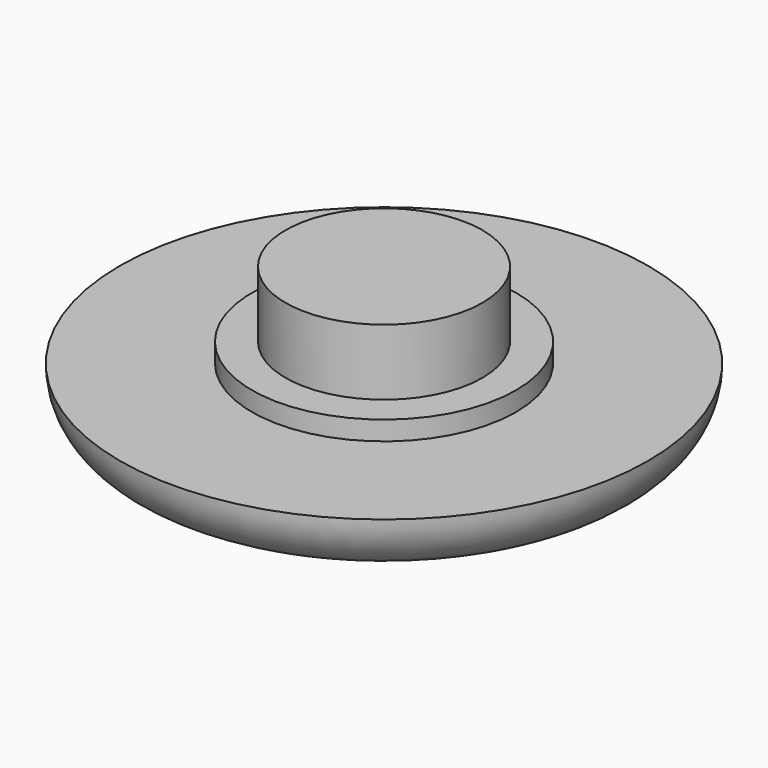
from build123d import *

# Parameters (mm, degrees)
F0_R      = 11
F0_R_2    = 5.5
F1_DEPTH  = 2.5
F0_R_3    = 4.1
F2_DEPTH  = 3.3
F3_DEPTH  = 6.05
F4_R      = 2.49999
F7_W      = 0.7752131331
F7_H      = 1.8432312268
F7_H_2    = 1.8120306982
F8_DEPTH  = 1
F9_W      = 0.005
F9_H      = 0.6400108426
F10_DEPTH = 0.1


# Not quite as in the source:
# - a fillet or chamfer is up to 0.001 mm smaller than in the source, because OpenCascade refuses the exact size


with BuildPart() as f1:
    # F0 (on Top) → F1 (new body)
    with BuildSketch(Plane.XY):
        Circle(F0_R)
        Circle(F0_R_2, mode=Mode.SUBTRACT)
    extrude(amount=F1_DEPTH)

    # F0 (on Top) → F2 (join, through all)
    with BuildSketch(Plane.XY):
        Circle(F0_R_2)
        Circle(F0_R_3, mode=Mode.SUBTRACT)
    extrude(amount=F2_DEPTH)

    # F0 (on Top) → F3 (join, through all)
    with BuildSketch(Plane.XY):
        Circle(F0_R_3)
    extrude(amount=F3_DEPTH)

    # F4 (radius 2.5 in the source; OpenCascade refuses exactly that, so slightly less here)
    f4_edges = [f1.edges().sort_by_distance(p)[0] for p in [
        (-11, 0, 0),
    ]]
    fillet(f4_edges, radius=F4_R)

    # F7 (on face) → F8 (cut)
    with BuildSketch(Plane(origin=(0, 0, 0), x_dir=(1, 0, 0), z_dir=(0, 0, -1))):
        with BuildLine():
            Line((-7.8377327815, 1.8120306982), (-7.8377327815, 0))
            Line((-7.8377327815, 0), (-7.0625196484, 0))
            Line((-7.0625196484, 0), (-7.0625196484, 1.1768199369))
            Line((-7.0625196484, 1.1768199369), (-6.6505126685, 1.1768199369))
            add(Edge.make_bspline(
                [(-5.6104951692, 0), (-5.6108483761, 1.1768199369), (-6.6505126685, 1.1768199369)],
                knots=[0.0003397316, 0.0003397316, 0.0003397316, 1, 1, 1], degree=2))
            Line((-5.6104951692, 0), (-4.8049398646, 0))
            add(Edge.make_bspline(
                [(-4.804881401, 0.0192003253), (-4.804881401, 0.0095761402), (-4.8049398646, 0)],
                knots=[0, 0, 0, 0.010664918, 0.010664918, 0.010664918], degree=2))
            add(Edge.make_bspline(
                [(-5.3000897905, 1.339622695), (-4.804881401, 0.8672146918), (-4.804881401, 0.0192003253)],
                knots=[0, 0, 0, 1, 1, 1], degree=2))
            add(Edge.make_bspline(
                [(-6.6905133461, 1.8120306982), (-5.79529818, 1.8120306982), (-5.3000897905, 1.339622695)],
                knots=[0, 0, 0, 1, 1, 1], degree=2))
            Line((-6.6905133461, 1.8120306982), (-7.8377327815, 1.8120306982))
        make_face()
        with BuildLine():
            Line((-7.0625196484, 0), (-7.8377327815, 0))
            Line((-7.8377327815, 0), (-7.8377327815, -1.8432312268))
            Line((-7.8377327815, -1.8432312268), (-6.8025152436, -1.8432312268))
            add(Edge.make_bspline(
                [(-5.318890109, -1.3632230948), (-5.832898817, -1.8432312268), (-6.8025152436, -1.8432312268)],
                knots=[0, 0, 0, 1, 1, 1], degree=2))
            add(Edge.make_bspline(
                [(-4.8049398646, 0), (-4.8103632617, -0.8883342102), (-5.318890109, -1.3632230948)],
                knots=[0.010664918, 0.010664918, 0.010664918, 1, 1, 1], degree=2))
            Line((-4.8049398646, 0), (-5.6104951692, 0))
            add(Edge.make_bspline(
                [(-5.6104950492, -0.0008000136), (-5.6104950492, -0.0003999388), (-5.6104951692, 0)],
                knots=[0, 0, 0, 0.0003397316, 0.0003397316, 0.0003397316], degree=2))
            add(Edge.make_bspline(
                [(-6.7305140238, -1.2032203841), (-5.6104950492, -1.2032203841), (-5.6104950492, -0.0008000136)],
                knots=[0, 0, 0, 1, 1, 1], degree=2))
            Line((-6.7305140238, -1.2032203841), (-7.0625196484, -1.2032203841))
            Line((-7.0625196484, -1.2032203841), (-7.0625196484, 0))
        make_face()
        Polygon((6.1985050109, 1.1672197742), (6.1985050109, 0), (6.973718144, 0), (6.973718144, 1.1672197742), (7.9657349501, 1.1672197742), (7.9657349501, 1.8120306982), (5.2056881912, 1.8120306982), (5.2056881912, 1.1672197742), align=None)
        with Locations((6.5861115774, -0.9216156134)):
            Rectangle(F7_W, F7_H)
        Polygon((3.2336547824, 1.1672197742), (3.2336547824, 0), (4.0088679155, 0), (4.0088679155, 1.1672197742), (5.0008847216, 1.1672197742), (5.0008847216, 1.8120306982), (2.2408379628, 1.8120306982), (2.2408379628, 1.1672197742), align=None)
        with Locations((3.6212613489, -0.9216156134)):
            Rectangle(F7_W, F7_H)
        with Locations((1.2908218682, 0.9060153491)):
            Rectangle(F7_W, F7_H_2)
        with Locations((1.2908218682, -0.9216156134)):
            Rectangle(F7_W, F7_H)
        Polygon((-4.5072763592, 1.8120306982), (-4.044849615, 0), (-3.3198281749, 0), (-3.7448634429, 1.8120306982), align=None)
        with BuildLine():
            Line((-3.3198281749, 0), (-4.044849615, 0))
            Line((-4.044849615, 0), (-3.5744605561, -1.8432312268))
            Line((-3.5744605561, -1.8432312268), (-2.6944456475, -1.8432312268))
            Line((-2.6944456475, -1.8432312268), (-2.2209338662, 0))
            Line((-2.2209338662, 0), (-2.868251717, 0))
            Line((-2.868251717, 0), (-2.9296496321, -0.2360039982))
            add(Edge.make_bspline(
                [(-3.0308513466, -0.6996118523), (-2.9768504318, -0.4008067902), (-2.9296496321, -0.2360039982)],
                knots=[0, 0, 0, 1, 1, 1], degree=2))
            add(Edge.make_bspline(
                [(-3.100052519, -1.140819327), (-3.0848522615, -0.9984169145), (-3.0308513466, -0.6996118523)],
                knots=[0, 0, 0, 1, 1, 1], degree=2))
            add(Edge.make_bspline(
                [(-3.2768555143, -0.1832031037), (-3.1544534406, -0.736012469), (-3.100052519, -1.140819327)],
                knots=[0, 0, 0, 1, 1, 1], degree=2))
            Line((-3.2768555143, -0.1832031037), (-3.3198281749, 0))
        make_face()
        with BuildLine():
            Line((-2.868251717, 0), (-3.3198281749, 0))
            Line((-3.3198281749, 0), (-3.2768555143, -0.1832031037))
            add(Edge.make_bspline(
                [(-3.2768555143, -0.1832031037), (-3.1544534406, -0.736012469), (-3.100052519, -1.140819327)],
                knots=[0, 0, 0, 1, 1, 1], degree=2))
            add(Edge.make_bspline(
                [(-3.100052519, -1.140819327), (-3.0848522615, -0.9984169145), (-3.0308513466, -0.6996118523)],
                knots=[0, 0, 0, 1, 1, 1], degree=2))
            add(Edge.make_bspline(
                [(-3.0308513466, -0.6996118523), (-2.9768504318, -0.4008067902), (-2.9296496321, -0.2360039982)],
                knots=[0, 0, 0, 1, 1, 1], degree=2))
            Line((-2.9296496321, -0.2360039982), (-2.868251717, 0))
        make_face()
        with BuildLine():
            Line((-2.3968406056, 1.8120306982), (-2.868251717, 0))
            Line((-2.868251717, 0), (-2.2209338662, 0))
            Line((-2.2209338662, 0), (-2.2024373122, 0.0720012198))
            add(Edge.make_bspline(
                [(-2.10963574, 0.4980084369), (-2.1696367565, 0.1992033748), (-2.2024373122, 0.0720012198)],
                knots=[0, 0, 0, 1, 1, 1], degree=2))
            add(Edge.make_bspline(
                [(-2.034434466, 0.9320157896), (-2.0496347235, 0.7968134991), (-2.10963574, 0.4980084369)],
                knots=[0, 0, 0, 1, 1, 1], degree=2))
            add(Edge.make_bspline(
                [(-1.9584331784, 0.5004084776), (-2.0248343034, 0.8216139192), (-2.034434466, 0.9320157896)],
                knots=[0, 0, 0, 1, 1, 1], degree=2))
            add(Edge.make_bspline(
                [(-1.8648315927, 0.0768013011), (-1.8920320535, 0.1792030359), (-1.9584331784, 0.5004084776)],
                knots=[0, 0, 0, 1, 1, 1], degree=2))
            Line((-1.8648315927, 0.0768013011), (-1.8450232571, 0))
            Line((-1.8450232571, 0), (-1.1934170931, 0))
            Line((-1.1934170931, 0), (-1.6648282044, 1.8120306982))
            Line((-1.6648282044, 1.8120306982), (-2.3968406056, 1.8120306982))
        make_face()
        with BuildLine():
            Line((-2.2024373122, 0.0720012198), (-2.2209338662, 0))
            Line((-2.2209338662, 0), (-1.8450232571, 0))
            Line((-1.8450232571, 0), (-1.8648315927, 0.0768013011))
            add(Edge.make_bspline(
                [(-1.8648315927, 0.0768013011), (-1.8920320535, 0.1792030359), (-1.9584331784, 0.5004084776)],
                knots=[0, 0, 0, 1, 1, 1], degree=2))
            add(Edge.make_bspline(
                [(-1.9584331784, 0.5004084776), (-2.0248343034, 0.8216139192), (-2.034434466, 0.9320157896)],
                knots=[0, 0, 0, 1, 1, 1], degree=2))
            add(Edge.make_bspline(
                [(-2.034434466, 0.9320157896), (-2.0496347235, 0.7968134991), (-2.10963574, 0.4980084369)],
                knots=[0, 0, 0, 1, 1, 1], degree=2))
            add(Edge.make_bspline(
                [(-2.10963574, 0.4980084369), (-2.1696367565, 0.1992033748), (-2.2024373122, 0.0720012198)],
                knots=[0, 0, 0, 1, 1, 1], degree=2))
        make_face()
        with BuildLine():
            Line((-1.1934170931, 0), (-1.8450232571, 0))
            Line((-1.8450232571, 0), (-1.3696232032, -1.8432312268))
            Line((-1.3696232032, -1.8432312268), (-0.487208254, -1.8432312268))
            Line((-0.487208254, -1.8432312268), (-0.0180294584, 0))
            Line((-0.0180294584, 0), (-0.7421344653, 0))
            Line((-0.7421344653, 0), (-0.7848132958, -0.1832031037))
            add(Edge.make_bspline(
                [(-0.8848149899, -0.6544110866), (-0.8296140548, -0.3632061532), (-0.7848132958, -0.1832031037)],
                knots=[0, 0, 0, 1, 1, 1], degree=2))
            add(Edge.make_bspline(
                [(-0.9648163453, -1.140819327), (-0.9400159251, -0.94561602), (-0.8848149899, -0.6544110866)],
                knots=[0, 0, 0, 1, 1, 1], degree=2))
            add(Edge.make_bspline(
                [(-1.0444176938, -0.6556111069), (-0.9920168061, -0.938415898), (-0.9648163453, -1.140819327)],
                knots=[0, 0, 0, 1, 1, 1], degree=2))
            add(Edge.make_bspline(
                [(-1.1320191779, -0.2360039982), (-1.0968185816, -0.3728063158), (-1.0444176938, -0.6556111069)],
                knots=[0, 0, 0, 1, 1, 1], degree=2))
            Line((-1.1320191779, -0.2360039982), (-1.1934170931, 0))
        make_face()
        with BuildLine():
            Line((-0.7421344653, 0), (-1.1934170931, 0))
            Line((-1.1934170931, 0), (-1.1320191779, -0.2360039982))
            add(Edge.make_bspline(
                [(-1.1320191779, -0.2360039982), (-1.0968185816, -0.3728063158), (-1.0444176938, -0.6556111069)],
                knots=[0, 0, 0, 1, 1, 1], degree=2))
            add(Edge.make_bspline(
                [(-1.0444176938, -0.6556111069), (-0.9920168061, -0.938415898), (-0.9648163453, -1.140819327)],
                knots=[0, 0, 0, 1, 1, 1], degree=2))
            add(Edge.make_bspline(
                [(-0.9648163453, -1.140819327), (-0.9400159251, -0.94561602), (-0.8848149899, -0.6544110866)],
                knots=[0, 0, 0, 1, 1, 1], degree=2))
            add(Edge.make_bspline(
                [(-0.8848149899, -0.6544110866), (-0.8296140548, -0.3632061532), (-0.7848132958, -0.1832031037)],
                knots=[0, 0, 0, 1, 1, 1], degree=2))
            Line((-0.7848132958, -0.1832031037), (-0.7421344653, 0))
        make_face()
        Polygon((-0.3200054213, 1.8120306982), (-0.7421344653, 0), (-0.0180294584, 0), (0.4432075085, 1.8120306982), align=None)
    extrude(amount=-F8_DEPTH, mode=Mode.SUBTRACT)

    # F9 (on face) → F10 (join)
    with BuildSketch(Plane(origin=(0, 0, 0), x_dir=(1, 0, 0), z_dir=(0, 0, -1))):
        with Locations((-7.0600196484, -1.5232258055)):
            Rectangle(F9_W, F9_H)
    extrude(amount=-F10_DEPTH)


solid = f1.part
